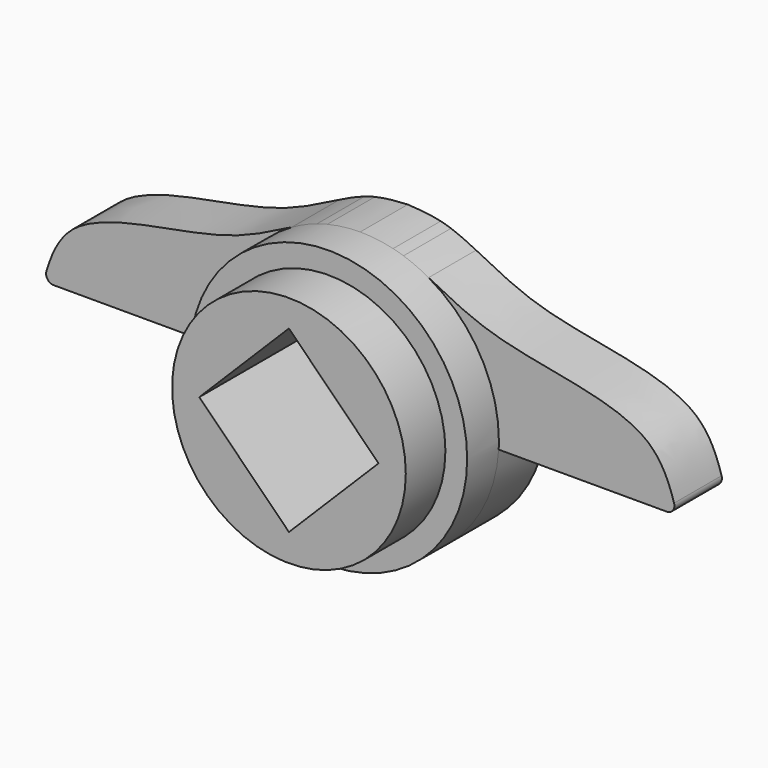
from build123d import *

# Parameters (mm, degrees)
F1_DEPTH = 3.81
F2_R     = 8.89
F3_DEPTH = 2.54
F4_R     = 7.493
F5_DEPTH = 3.175
F6_R     = 0.4911819864


with BuildPart() as f1:
    # F0 (on Front) → F1 (new body)
    with BuildSketch(Plane.XZ):
        with BuildLine():
            ThreePointArc((8.8754738465, -0.508), (8.8863677196, -0.2541038219), (8.89, 0))
            ThreePointArc((8.89, 0), (7.6804215502, 4.4769660275), (4.3808380628, 7.7356549734))
            add(Edge.make_bspline(
                [(2.7757389763, 8.4455534535), (3.2888417453, 8.2703062234), (3.8159102337, 8.0198976132), (4.3808380628, 7.7356549734)],
                knots=[0.1783179795, 0.1783179795, 0.1783179795, 0.1783179795, 0.2655314771, 0.2655314771, 0.2655314771, 0.2655314771], degree=3))
            ThreePointArc((2.7757389763, 8.4455534535), (2.4438853282, 8.5474864435), (2.1083049646, 8.6363852494))
            add(Edge.make_bspline(
                [(0, 8.89), (0.577506035, 8.8570186599), (1.3119112895, 8.8227589155), (2.1083049646, 8.6363852494)],
                knots=[0, 0, 0, 0, 0.1399319156, 0.1399319156, 0.1399319156, 0.1399319156], degree=3))
            add(Edge.make_bspline(
                [(0, 8.89), (-0.577506035, 8.8570186599), (-1.3119112895, 8.8227589155), (-2.1083049646, 8.6363852494)],
                knots=[0, 0, 0, 0, 0.1399319156, 0.1399319156, 0.1399319156, 0.1399319156], degree=3))
            ThreePointArc((-2.1083049646, 8.6363852494), (-2.4438853282, 8.5474864435), (-2.7757389763, 8.4455534535))
            add(Edge.make_bspline(
                [(-2.7757389763, 8.4455534535), (-3.2888417453, 8.2703062234), (-3.8159102337, 8.0198976132), (-4.3808380628, 7.7356549734)],
                knots=[0.1783179795, 0.1783179795, 0.1783179795, 0.1783179795, 0.2655314771, 0.2655314771, 0.2655314771, 0.2655314771], degree=3))
            ThreePointArc((-4.3808380628, 7.7356549734), (-7.8052490793, 4.255606515), (-8.8754738465, -0.508))
            Line((-8.8754738465, -0.508), (-5.2194662387, -0.508))
            Line((-5.2194662387, -0.508), (-5.7473639175, 0.0198976788))
            Line((-5.7473639175, 0.0198976788), (0, 5.7672615963))
            Line((0, 5.7672615963), (5.7473639175, 0.0198976788))
            Line((5.7473639175, 0.0198976788), (5.2194662387, -0.508))
            Line((5.2194662387, -0.508), (8.8754738465, -0.508))
        make_face()
        with BuildLine():
            ThreePointArc((4.3808380628, 7.7356549734), (7.6804215502, 4.4769660275), (8.89, 0))
            ThreePointArc((8.89, 0), (8.8863677196, -0.2541038219), (8.8754738465, -0.508))
            Line((8.8754738465, -0.508), (20.32, -0.508))
            add(Edge.make_bspline(
                [(4.3808380628, 7.7356549734), (5.5525412949, 7.1461141461), (9.398567587, 5.0276978273), (19.2176653381, 4.6545545686), (20.0494547253, 0.2736910266), (20.32, -0.508)],
                knots=[0.2655314771, 0.2655314771, 0.2655314771, 0.2655314771, 0.4464188962, 0.7868227895, 1, 1, 1, 1], degree=3))
        make_face()
        with BuildLine():
            ThreePointArc((-8.8754738465, -0.508), (0, -8.89), (8.8754738465, -0.508))
            Line((8.8754738465, -0.508), (5.2194662387, -0.508))
            Line((5.2194662387, -0.508), (0, -5.7274662387))
            Line((0, -5.7274662387), (-5.2194662387, -0.508))
            Line((-5.2194662387, -0.508), (-8.8754738465, -0.508))
        make_face()
        with BuildLine():
            Line((-20.32, -0.508), (-8.8754738465, -0.508))
            ThreePointArc((-8.8754738465, -0.508), (-7.8052490793, 4.255606515), (-4.3808380628, 7.7356549734))
            add(Edge.make_bspline(
                [(-4.3808380628, 7.7356549734), (-5.5525412949, 7.1461141461), (-9.398567587, 5.0276978273), (-19.2176653381, 4.6545545686), (-20.0494547253, 0.2736910266), (-20.32, -0.508)],
                knots=[0.2655314771, 0.2655314771, 0.2655314771, 0.2655314771, 0.4464188962, 0.7868227895, 1, 1, 1, 1], degree=3))
        make_face()
    extrude(amount=F1_DEPTH)

    # F2 (on face) → F3 (join)
    with BuildSketch(Plane.XZ.offset(3.81)):
        Circle(F2_R)
        Polygon((-5.7473639175, 0.0198976788), (0, 5.7672615963), (5.7473639175, 0.0198976788), (0, -5.7274662387), align=None, mode=Mode.SUBTRACT)
    extrude(amount=F3_DEPTH)

    # F4 (on face) → F5 (join)
    with BuildSketch(Plane.XZ.offset(6.35)):
        Circle(F4_R)
        Polygon((0, -5.7274662387), (-5.7473639175, 0.0198976788), (0, 5.7672615963), (5.7473639175, 0.0198976788), align=None, mode=Mode.SUBTRACT)
    extrude(amount=F5_DEPTH)

    # F6
    f6_edges = [f1.edges().sort_by_distance(p)[0] for p in [
        (20.32, -1.905, -0.508),
        (-20.32, -1.905, -0.508),
    ]]
    fillet(f6_edges, radius=F6_R)


solid = f1.part
